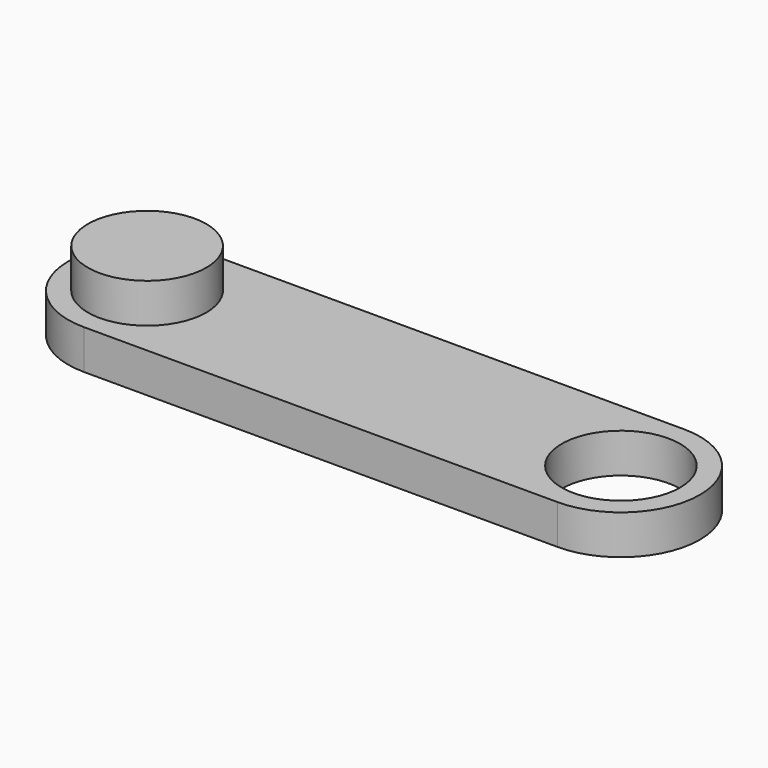
from build123d import *

# Parameters (mm, degrees)
F2_DEPTH = 12.7
F3_R     = 19.05
F4_DEPTH = 12.7
F5_DEPTH = 12.7


# Not quite as in the source:
# - a variable given as a bare number and used for a length is read in inches; the dataset says mm whatever the document's units were


with BuildPart() as f2:
    # F1 (on Top) → F2 (new body)
    with BuildSketch(Plane.XY):
        with BuildLine():
            Line((-76.2, -25.4), (76.2, -25.4))
            ThreePointArc((76.2, -25.4), (101.6, 0), (76.2, 25.4))
            Line((76.2, 25.4), (-76.2, 25.4))
            ThreePointArc((-76.2, 25.4), (-101.6, 0), (-76.2, -25.4))
        make_face()
    extrude(amount=F2_DEPTH)

    # F3 (on face) → F4 (join)
    with BuildSketch(Plane.XY.offset(12.7)):
        with Locations((-76.2, 0)):
            Circle(F3_R)
    extrude(amount=F4_DEPTH)

    # F3 (on face) → F5 (cut)
    with BuildSketch(Plane.XY.offset(12.7)):
        with Locations((76.2, 0)):
            Circle(F3_R)
    extrude(amount=-F5_DEPTH, mode=Mode.SUBTRACT)


solid = f2.part
